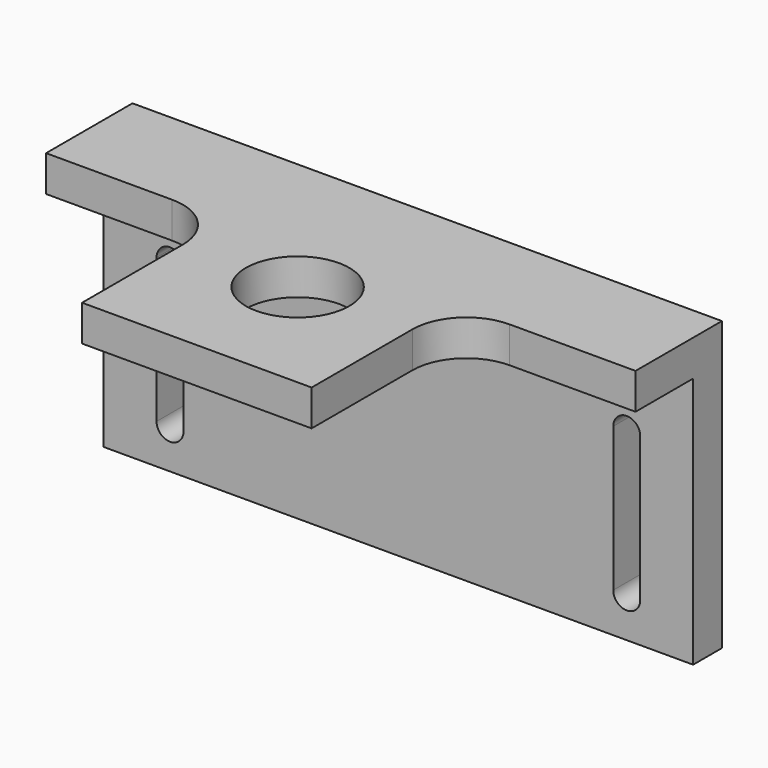
from build123d import *

# Parameters (mm, degrees)
F0_W     = 104
F0_H     = 50.8
F1_DEPTH = 6.35
F2_W     = 104
F2_H     = 44.45
F3_DEPTH = 6.35
F6_D     = 18.25625
F8_DEPTH = 50.801
F9_DEPTH = 50.801


# Not quite as in the source:
# - a length typed as a fraction of an inch, garbled in the dataset ("3 / 203.2 mm" for 3/8 in), is restored


with BuildPart() as f1:
    # F0 (on Front) → F1 (new body)
    with BuildSketch(Plane.XZ):
        Rectangle(F0_W, F0_H)
    extrude(amount=F1_DEPTH)

    # F2 (on face) → F3 (join)
    with BuildSketch(Plane.XY.offset(25.4)):
        with Locations((0, -28.575)):
            Rectangle(F2_W, F2_H)
    extrude(amount=-F3_DEPTH)

    # F6 (through all)
    with Locations(Plane.XY.offset(25.4)):
        with Locations((0, -28.575)):
            Hole(F6_D / 2)

    # F7 (on face) → F8 (cut, through all)
    with BuildSketch(Plane.XY.offset(25.4)):
        with BuildLine():
            Line((-29.775, -19.05), (-52, -19.05))
            Line((-52, -19.05), (-52, -50.8))
            Line((-52, -50.8), (-20.25, -50.8))
            Line((-20.25, -50.8), (-20.25, -28.575))
            ThreePointArc((-20.25, -28.575), (-23.0398079092, -21.8398079092), (-29.775, -19.05))
        make_face()
        with BuildLine():
            Line((20.25, -28.575), (20.25, -50.8))
            Line((20.25, -50.8), (52, -50.8))
            Line((52, -50.8), (52, -19.05))
            Line((52, -19.05), (29.775, -19.05))
            ThreePointArc((29.775, -19.05), (23.0398079092, -21.8398079092), (20.25, -28.575))
        make_face()
    extrude(amount=-F8_DEPTH, mode=Mode.SUBTRACT)

    # F4 (on face) → F9 (cut, through all)
    with BuildSketch(Plane(origin=(0, 0, 0), x_dir=(-1, 0, 0), z_dir=(0, 1, 0))):
        with BuildLine():
            ThreePointArc((37.9072132349, -18.4), (40.2884632349, -20.78125), (42.6697132349, -18.4))
            Line((42.6697132349, -18.4), (42.6697132349, 7.05))
            ThreePointArc((42.6697132349, 7.05), (40.2884632349, 9.43125), (37.9072132349, 7.05))
            Line((37.9072132349, 7.05), (37.9072132349, -18.4))
        make_face()
        with BuildLine():
            ThreePointArc((-42.6697132349, -18.4), (-40.2884632349, -20.78125), (-37.9072132349, -18.4))
            Line((-37.9072132349, -18.4), (-37.9072132349, 7.05))
            ThreePointArc((-37.9072132349, 7.05), (-40.2884632349, 9.43125), (-42.6697132349, 7.05))
            Line((-42.6697132349, 7.05), (-42.6697132349, -18.4))
        make_face()
    extrude(amount=-F9_DEPTH, mode=Mode.SUBTRACT)


solid = f1.part
